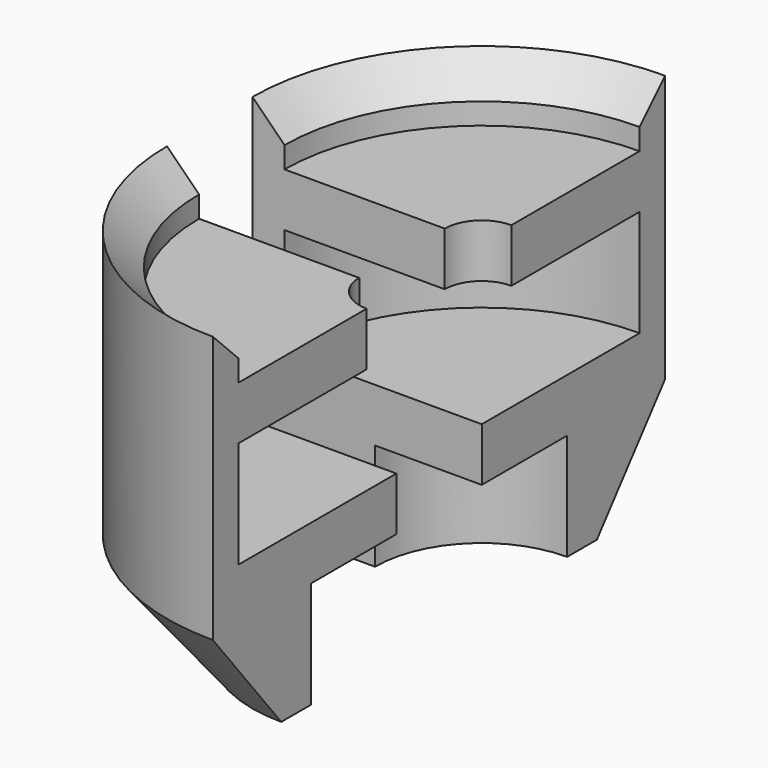
from build123d import *

# Parameters (mm, degrees)
F1_ANGLE = 90
F2_SIZE  = 7.61999


# Not quite as in the source:
# - a fillet or chamfer is up to 0.001 mm smaller than in the source, because OpenCascade refuses the exact size


with BuildPart() as f1:
    # F0 (on Front) → F1 (revolve)
    with BuildSketch(Plane.XZ):
        Polygon((-8.8121203113, 0), (0, 0), (0, 25.4), (25.4, 25.4), (25.4, 38.1), (-21.5121203113, 38.1), (-21.5121203113, 63.5), (16.5878796887, 63.5), (16.5878796887, 76.2), (-21.5121203113, 76.2), (-21.5121203113, 88.9), (-29.1321203113, 88.9), (-29.1321203113, 25.4), align=None)
    revolve(axis=Axis((25.4, 0, 31.75), (0, 0, 1)), revolution_arc=F1_ANGLE)

    # F2 (size 7.62 in the source; OpenCascade refuses exactly that, so slightly less here)
    f2_edges = [f1.edges().sort_by_distance(p)[0] for p in [
        (-7.771878, -33.171878, 88.9),
    ]]
    chamfer(f2_edges, length=F2_SIZE)


with BuildPart() as f4_1:
    # F4: instance of F1
    add(f1.part.mirror(Plane(origin=(-8.2304534557, 12.7, 42.1908362941), x_dir=(-1, 0, 0), z_dir=(0, 1, 0))))


solid = Compound([f1.part, f4_1.part])
